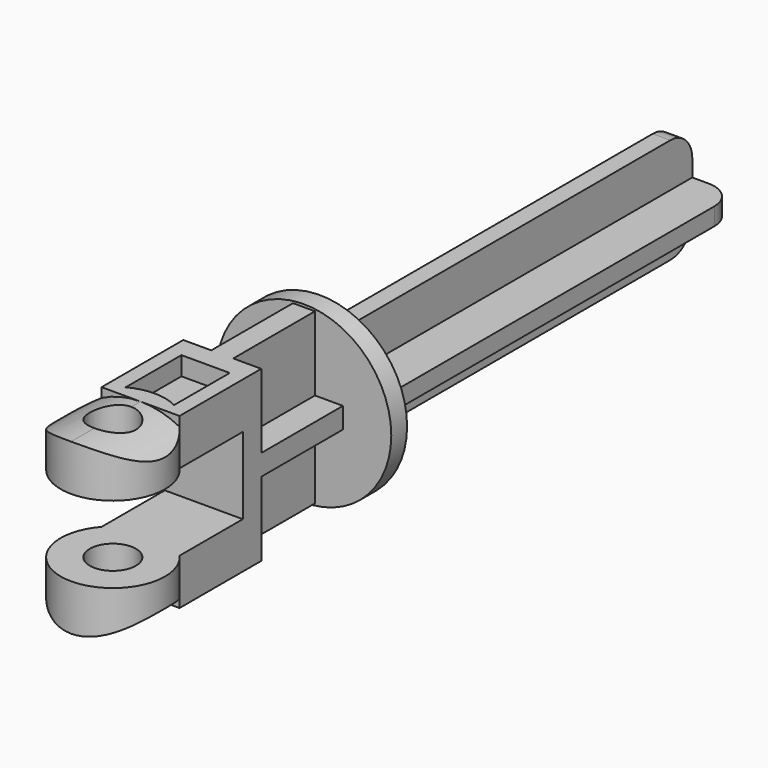
from build123d import *

# Parameters (mm, degrees)
F0_R             = 7.95
F1_DEPTH         = 1.8
F3_DEPTH         = 41.4
F5_W             = 7.1
F5_H             = 15.4
F6_DEPTH         = 9.3
F7_W             = 2.55
F7_H             = 9.3
F8_DEPTH         = 6.75
F8_COPIES2_COUNT = 2
F10_DEPTH        = 12.7
F11_R            = 4.75
F12_DEPTH        = 7.7
F12_DEPTH_BACK   = 7.7
F15_DEPTH        = 8.2
F16_W            = 3.7673835978
F16_H            = 7
F16_W_2          = 9.5
F16_W_3          = 4.3988060828
F17_DEPTH        = 15.4
F18_R            = 2.1
F19_DEPTH        = 7.951
F19_DEPTH_BACK   = 25
F20_R            = 2.5
F22_R            = 2.1
F23_DEPTH        = 25


# Not quite as in the source:
# - a feature of the source that left no trace in its solid (it failed there, or was rolled back) is left out
# - a pattern or mirror of a feature is missing from the dataset's text; its kind, count and spacing are read off the source's solid


with BuildPart() as f1:
    # F0 (on Front) → F1 (new body)
    with BuildSketch(Plane.XZ):
        Circle(F0_R)
    extrude(amount=-F1_DEPTH)

    # F2 (on face) → F3 (join)
    with BuildSketch(Plane(origin=(0, 1.8, 0), x_dir=(-1, 0, 0), z_dir=(0, 1, 0))):
        Polygon((0.8, 0.8), (0.8, 4.8), (-0.8, 4.8), (-0.8, 0.8), (-4.8, 0.8), (-4.8, -0.8), (-0.8, -0.8), (-0.8, -4.8), (0.8, -4.8), (0.8, -0.8), (4.8, -0.8), (4.8, 0.8), align=None)
    extrude(amount=F3_DEPTH)

    # F5 (on Front) → F6 (join)
    with BuildSketch(Plane.XZ):
        Rectangle(F5_W, F5_H)
    extrude(amount=F6_DEPTH)

    # F7 (on face) → F8 (cut)
    with BuildSketch(Plane.XY.offset(7.7)):
        with Locations((-2.275, -4.65)):
            Rectangle(F7_W, F7_H)
    f8 = extrude(amount=-F8_DEPTH, mode=Mode.SUBTRACT)

    # F8_copies: F8 across plane
    add(f8.mirror(Plane(origin=(0, 0, 0), x_dir=(-1, 0, 0), z_dir=(0, 0, -1))), mode=Mode.SUBTRACT)

    # F8_copies1: F8 across plane
    add(f8.mirror(Plane(origin=(0, 0, 0), x_dir=(0, 0, 1), z_dir=(1, 0, 0))), mode=Mode.SUBTRACT)

    # F8_copies2: F8 ×2 about axis
    f8_copies2_axis = Axis((0, 0, 0), (0, 1, 0))
    for i in range(1, F8_COPIES2_COUNT):
        add(f8.rotate(f8_copies2_axis, i * 360 / F8_COPIES2_COUNT), mode=Mode.SUBTRACT)

    # F9 (on offset) → F10 (join)
    with BuildSketch(Plane.XZ.offset(9.3)):
        Polygon((-1, 7.7), (-3.55, 7.7), (-3.55, -7.7), (3.55, -7.7), (3.55, -0.95), (3.55, 0.95), (3.55, 7.7), (1, 7.7), align=None)
    extrude(amount=F10_DEPTH)

    # F11 (on Top) → F12 (join, two sides)
    with BuildSketch(Plane.XY) as f12_sk:
        with Locations((0, -21.75)):
            Circle(F11_R)
    extrude(amount=F12_DEPTH)
    extrude(f12_sk.sketch, amount=-F12_DEPTH_BACK)

    # F14 (on offset) → F15 (cut)
    with BuildSketch(Plane.XZ.offset(26.8)):
        with BuildLine():
            ThreePointArc((0, 7.7), (5.4447222151, 5.4447222151), (7.7, 0))
            Line((7.7, 0), (7.7, 7.7))
            Line((7.7, 7.7), (0, 7.7))
        make_face()
        with BuildLine():
            ThreePointArc((-7.7, 0), (-5.4447222151, 5.4447222151), (0, 7.7))
            Line((0, 7.7), (-7.7, 7.7))
            Line((-7.7, 7.7), (-7.7, 0))
        make_face()
        with BuildLine():
            Line((-7.7, -7.7), (0, -7.7))
            ThreePointArc((0, -7.7), (-5.4447222151, -5.4447222151), (-7.7, 0))
            Line((-7.7, 0), (-7.7, -7.7))
        make_face()
        with BuildLine():
            Line((7.7, -7.7), (7.7, 0))
            ThreePointArc((7.7, 0), (5.4447222151, -5.4447222151), (0, -7.7))
            Line((0, -7.7), (7.7, -7.7))
        make_face()
    extrude(amount=-F15_DEPTH, mode=Mode.SUBTRACT)

    # F16 (on offset) → F17 (cut)
    with BuildSketch(Plane.XZ.offset(26.8)):
        with Locations((-6.6336917989, 0)):
            Rectangle(F16_W, F16_H)
        Rectangle(F16_W_2, F16_H)
        with Locations((6.9494030414, 0)):
            Rectangle(F16_W_3, F16_H)
    extrude(amount=-F17_DEPTH, mode=Mode.SUBTRACT)

    # F18 (on Top) → F19 (cut, two sides)
    with BuildSketch(Plane.XY) as f19_sk:
        with Locations((0, -21.75)):
            Circle(F18_R)
    extrude(amount=-F19_DEPTH, mode=Mode.SUBTRACT)
    extrude(f19_sk.sketch, amount=F19_DEPTH_BACK, mode=Mode.SUBTRACT)

    # F20
    f20_edges = [f1.edges().sort_by_distance(p)[0] for p in [
        (0, 43.2, 4.8),
        (4.8, 43.2, 0),
        (0, 43.2, -4.8),
        (-4.8, 43.2, 0),
    ]]
    fillet(f20_edges, radius=F20_R)

    # F22 (on offset) → F23 (cut)
    with BuildSketch(Plane.XY.offset(-6)):
        with Locations((0, -21.75)):
            Circle(F22_R)
        with BuildLine():
            ThreePointArc((-2.2, -17.540190028), (0, -17), (2.2, -17.540190028))
            Line((2.2, -17.540190028), (2.2, -11.2))
            Line((2.2, -11.2), (-2.2, -11.2))
            Line((-2.2, -11.2), (-2.2, -17.540190028))
        make_face()
    f23 = extrude(amount=-F23_DEPTH, mode=Mode.SUBTRACT)

    # F23_copies: F23 across plane
    add(f23.mirror(Plane.XY), mode=Mode.SUBTRACT)


solid = f1.part
